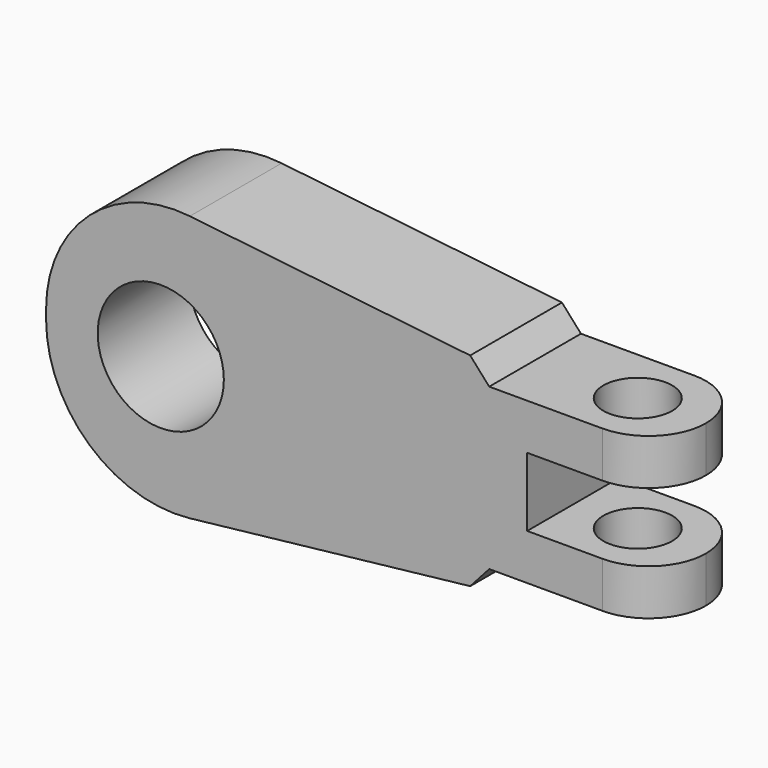
from build123d import *

# Parameters (mm, degrees)
F1_DEPTH     = 10
F3_DEPTH     = 25
F4_R         = 3
F5_DEPTH     = 12.5
F6_R         = 4.99999
F7_R         = 11.2793724654
F8_W         = 12.0593691245
F8_H         = 3
F9_DEPTH     = 25
F10_T4_DEPTH = 35.7540736123
F10_T9_DEPTH = 35.7540736123


# Not quite as in the source:
# - a fillet or chamfer that OpenCascade refuses, or shapes differently, is made with other operations: its cross-section is extruded or revolved along the edge and cut away or added
# - a fillet or chamfer is up to 0.001 mm smaller than in the source, because OpenCascade refuses the exact size


with BuildPart() as f1:
    # F0 (on Front) → F1 (new body)
    with BuildSketch(Plane.XZ):
        Polygon((-29.8706907779, 13), (-29.8706907779, 0), (-29.8706907779, -13), (23.6637946218, -7), (23.6637946218, 0), (23.6637946218, 7), align=None)
    extrude(amount=F1_DEPTH)

    # F2 (on face) → F3 (cut)
    with BuildSketch(Plane.XZ.offset(10)):
        with BuildLine():
            ThreePointArc((-25.3706907779, 0), (-19.8706907779, -5.5), (-14.3706907779, 0))
            ThreePointArc((-14.3706907779, 0), (-19.8706907779, 5.5), (-25.3706907779, 0))
        make_face()
    extrude(amount=-F3_DEPTH, mode=Mode.SUBTRACT)

    # F4 (on Top) → F5 (cut, symmetric)
    with BuildSketch(Plane.XY):
        with Locations((17.7213400602, -4.9999998882)):
            Circle(F4_R)
    extrude(amount=F5_DEPTH, both=True, mode=Mode.SUBTRACT)

    # F6 (radius 5 in the source; OpenCascade refuses exactly that, so slightly less here)
    f6_edges = [f1.edges().sort_by_distance(p)[0] for p in [
        (23.663795, -10, 0),
        (23.663795, 0, 0),
    ]]
    fillet(f6_edges, radius=F6_R)

    # F7
    f7_edges = [f1.edges().sort_by_distance(p)[0] for p in [
        (-29.870691, -5, 13),
        (-29.870691, -5, -13),
    ]]
    fillet(f7_edges, radius=F7_R)

    # F8 (on Front) → F9 (cut)
    with BuildSketch(Plane.XZ):
        Polygon((12.0786419138, 3), (12.0786419138, 0), (24.1380110383, 0), (24.2066532373, 3), align=None)
        with Locations((18.1083264761, -1.5)):
            Rectangle(F8_W, F8_H)
        Polygon((25.2308808267, -17.6116619259), (24.1380110383, -7), (12.0786419138, -7), (12.0786419138, -17.6116619259), align=None)
        Polygon((12.0786419138, 14.7170173004), (12.0786419138, 7), (24.2066532373, 7), (23.395627737, 15.3522975743), align=None)
    extrude(amount=F9_DEPTH, mode=Mode.SUBTRACT)

    # F10: chamfer of 5 on 2 edges, made by hand


with BuildPart() as f10_tool2:
    # F10_s3 → F10_t4 (new body)
    with BuildSketch(Plane.XZ.offset(22.8770368062)):
        Polygon((12.0786419138, -3.29843251), (7.1097524238, -8.8553321741), (12.0786419138, -8.29843251), align=None)
    extrude(amount=-F10_T4_DEPTH)

    split(bisect_by=Plane.XY.offset(-7), keep=Keep.BOTTOM)


with BuildPart() as f1_1:
    add(f1.part)

    # F10_t1: cut F10_tool2
    add(f10_tool2.part, mode=Mode.SUBTRACT)


with BuildPart() as f10_tool7:
    # F10_s8 → F10_t9 (new body)
    with BuildSketch(Plane.XZ.offset(-12.8770368062)):
        Polygon((7.1097524238, 8.8553321741), (12.0786419138, 3.29843251), (12.0786419138, 8.29843251), align=None)
    extrude(amount=F10_T9_DEPTH)

    split(bisect_by=Plane.XY.offset(7), keep=Keep.TOP)


with BuildPart() as f1_2:
    add(f1_1.part)

    # F10_t6: cut F10_tool7
    add(f10_tool7.part, mode=Mode.SUBTRACT)


solid = f1_2.part
